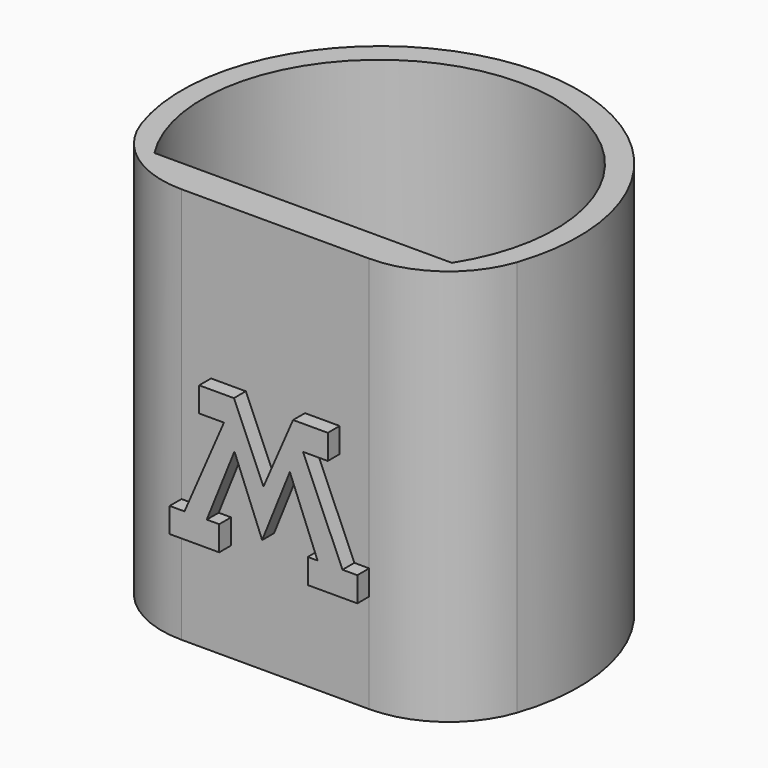
from build123d import *

# Parameters (mm, degrees)
F1_DEPTH = 101.6
F3_DEPTH = 95.25
F4_R     = 25.4
F6_DEPTH = 3.81


# Not quite as in the source:
# - a feature names something its author has since deleted; it is built from what else it names


with BuildPart() as f1:
    # F0 (on Top) → F1 (new body)
    with BuildSketch(Plane.XY):
        with BuildLine():
            ThreePointArc((33.8925523579, 0), (-4.2074476421, 84.4010416505), (-42.3074476421, 0))
            Line((-42.3074476421, 0), (33.8925523579, 0))
        make_face()
    extrude(amount=F1_DEPTH)

    # F2 (on face) → F3 (cut)
    with BuildSketch(Plane.XY.offset(101.6)):
        with BuildLine():
            ThreePointArc((33.8925523579, 8.89), (-4.2074476421, 78.3858036913), (-42.3074476421, 8.89))
            Line((-42.3074476421, 8.89), (33.8925523579, 8.89))
        make_face()
    extrude(amount=-F3_DEPTH, mode=Mode.SUBTRACT)

    # F4
    f4_edges = [f1.edges().sort_by_distance(p)[0] for p in [
        (-42.307448, 0, 50.8),
        (33.892552, 0, 50.8),
    ]]
    fillet(f4_edges, radius=F4_R)

    # F5 (on face) → F6 (join)
    with BuildSketch(Plane.XZ):
        Polygon((-28.2470590334, 31.75), (-28.2470590334, 25.4), (-15.5470590334, 25.4), (-15.5470590334, 31.75), (-18.7367527627, 31.75), (-11.6416137586, 49.4294089978), (-4.5464747545, 31.75), (2.5486642496, 49.4294089978), (9.6438032537, 31.75), (7.1321637492, 31.75), (7.1321637492, 25.4), (19.8321637492, 25.4), (19.8321637492, 31.75), (16.0221637492, 31.75), (5.9138143828, 55.0519585676), (12.2638143828, 55.0519585676), (12.2638143828, 61.4019585676), (3.3738143828, 61.4019585676), (-4.2074476421, 43.9254896419), (-11.7887096669, 61.4019585676), (-20.6787096669, 61.4019585676), (-20.6787096669, 55.0519585676), (-14.3287096669, 55.0519585676), (-24.4370590334, 31.75), align=None)
    extrude(amount=F6_DEPTH)


solid = f1.part
